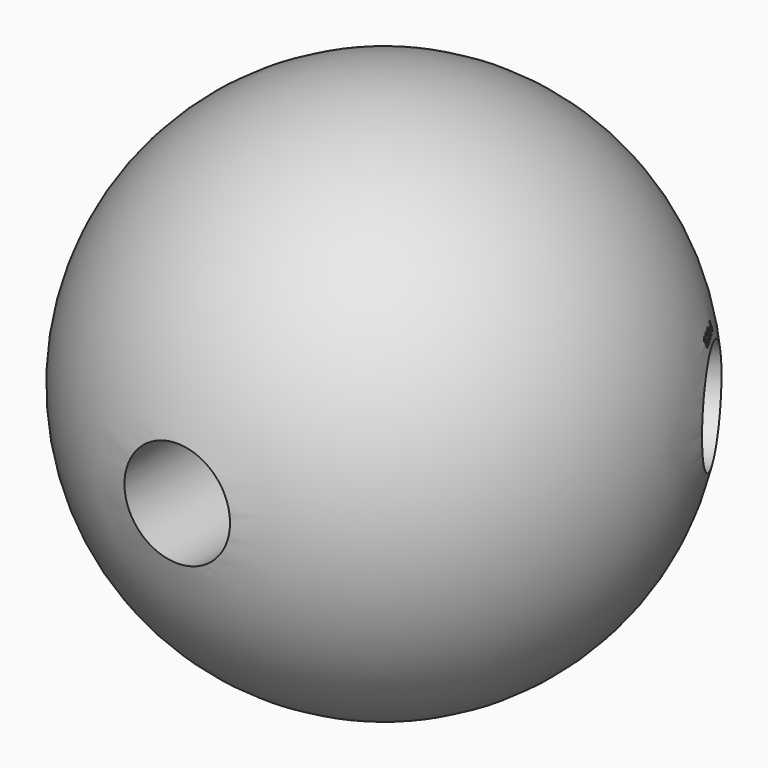
from build123d import *

# Parameters (mm, degrees)
F4_R          = 3.175
F5_DEPTH      = 25.4
F8_ANGLE      = 119.9
F9_ANGLE      = -120.7
F10_ANGLE     = 120.2
F12_TEXT_SIZE = 1.2863188102
F13_DEPTH     = 2.0828
F15_ANGLE     = -120.4
F17_TEXT_SIZE = 0.831208955
F18_DEPTH     = 2.2098


# Not quite as in the source:
# - Text() gives the source's letters only with a copy of the font that has no kerning and outlines rounded to 1/6400 em; it was checked with that copy


with BuildPart() as f2:
    # F0 (on Front) → F2 (revolve)
    with BuildSketch(Plane.XZ):
        with BuildLine():
            Line((0, -15.875), (0, 15.875))
            ThreePointArc((0, 15.875), (-15.875, 0), (0, -15.875))
        make_face()
    revolve(axis=Axis((0, 0, 0), (0, 0, 1)))

    # F12 (on offset) → F13 (cut)
    with BuildSketch(Plane(origin=(-14.44479762, 8.407072972, 0), x_dir=(-0.5030199466, -0.864274802, 0), z_dir=(-0.864274802, 0.5030199466, 0))):
        with Locations((-1.5270224467, 3.6735176109)):
            Text('120.2', F12_TEXT_SIZE, font='Open Sans', font_style=FontStyle.BOLD, text_align=(TextAlign.LEFT, TextAlign.BOTTOM))
    extrude(amount=-F13_DEPTH, mode=Mode.SUBTRACT)


with BuildPart() as f5:
    # F4 (on offset) → F5 (new body)
    with BuildSketch(Plane.XZ.offset(6.35)):
        Circle(F4_R)
    extrude(amount=F5_DEPTH)


with BuildPart() as f8_1:
    # F8: copy of F5
    add(f5.part.rotate(Axis((4.3243672699, 0, 0), (-1, 0, 0)), F8_ANGLE))


with BuildPart() as f9_1:
    # F9: copy of F5
    add(f5.part.rotate(Axis((4.3243672699, 0, 0), (-1, 0, 0)), F9_ANGLE))


with BuildPart() as f10_1:
    # F10: copy of F5
    add(f5.part.rotate(Axis((0, 0, 6.8211313337), (0, 0, -1)), F10_ANGLE))


with BuildPart() as f2_1:
    add(f2.part)

    # F14: cut F10_1
    add(f10_1.part, mode=Mode.SUBTRACT)

    # F17 (on offset) → F18 (cut)
    with BuildSketch(Plane(origin=(14.6563497754, 8.5988293402, 0), x_dir=(-0.5060337641, 0.8625136692, 0), z_dir=(0.8625136692, 0.5060337641, 0))):
        with Locations((-1.1224457921, 3.4937013406)):
            Text('120.4', F17_TEXT_SIZE, font='Open Sans', font_style=FontStyle.BOLD, text_align=(TextAlign.LEFT, TextAlign.BOTTOM))
    extrude(amount=-F18_DEPTH, mode=Mode.SUBTRACT)


with BuildPart() as f15_1:
    # F15: copy of F5
    add(f5.part.rotate(Axis((0, 0, 6.8211313337), (0, 0, -1)), F15_ANGLE))


with BuildPart() as f2_2:
    add(f2_1.part)

    # F19: cut F15_1
    add(f15_1.part, mode=Mode.SUBTRACT)

    # F20: cut F5
    add(f5.part, mode=Mode.SUBTRACT)


solid = f2_2.part
